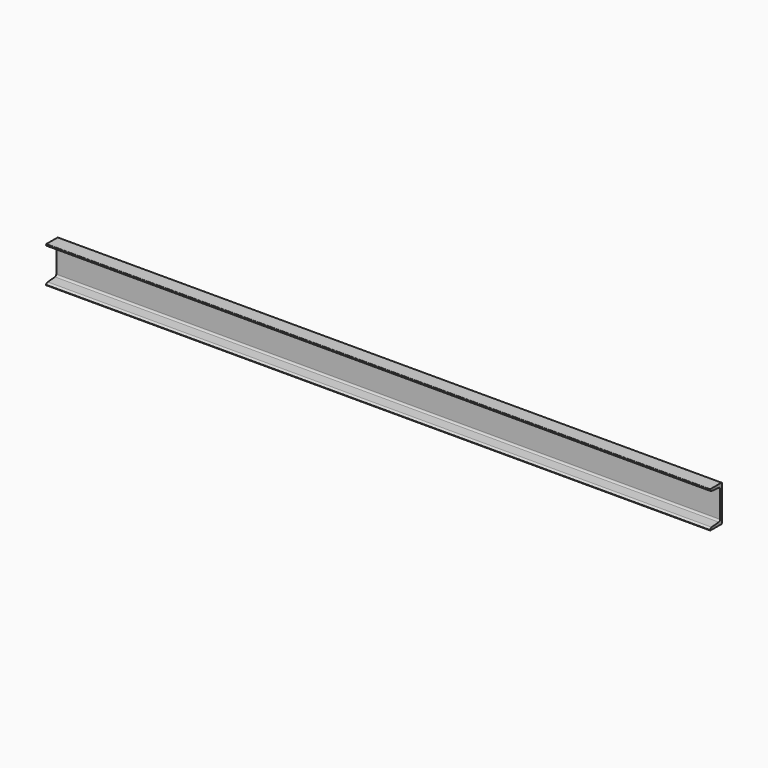
from build123d import *

# Parameters (mm, degrees)
F1_DEPTH    = 924
F2_T1_DEPTH = 1877.7738168108


# Not quite as in the source:
# - a fillet or chamfer that OpenCascade refuses, or shapes differently, is made with other operations: its cross-section is extruded or revolved along the edge and cut away or added


with BuildPart() as f1:
    # F0 (on Right) → F1 (new body, symmetric)
    with BuildSketch(Plane.YZ):
        with BuildLine():
            ThreePointArc((-20.915, -48.8), (-20.3292135624, -50.2142135624), (-18.915, -50.8))
            Line((-18.915, -50.8), (18.915, -50.8))
            ThreePointArc((18.915, -50.8), (20.3292135624, -50.2142135624), (20.915, -48.8))
            Line((20.915, -48.8), (20.915, 48.8))
            ThreePointArc((20.915, 48.8), (20.3292135624, 50.2142135624), (18.915, 50.8))
            Line((18.915, 50.8), (-18.915, 50.8))
            ThreePointArc((-18.915, 50.8), (-20.3292135624, 50.2142135624), (-20.915, 48.8))
            Line((-20.915, 48.8), (-20.915, 44.8355484375))
            Line((-20.915, 44.8355484375), (10.0807787137, 42.1237691829))
            ThreePointArc((10.0807787137, 42.1237691829), (13.3313866841, 40.5207467305), (14.645, 37.1427956924))
            Line((14.645, 37.1427956924), (14.645, -37.1427956924))
            ThreePointArc((14.645, -37.1427956924), (13.3313866841, -40.5207467305), (10.0807787137, -42.1237691829))
            Line((10.0807787137, -42.1237691829), (-20.915, -44.8355484375))
            Line((-20.915, -44.8355484375), (-20.915, -48.8))
        make_face()
    extrude(amount=F1_DEPTH, both=True)

    # F2: fillet of radius 7 on 2 edges, made by hand

    # F2_s2 → F2_t1 (cut)
    with BuildSketch(Plane.YZ.offset(-938.8869084054)):
        with BuildLine():
            ThreePointArc((-20.915, -48.8), (-18.5934823683, -45.7054865005), (-14.9828963102, -44.3165566138))
            Line((-14.9828963102, -44.3165566138), (-14.9950981142, -44.177089356))
            Line((-14.9950981142, -44.177089356), (-20.927201804, -44.6960811798))
            Line((-20.927201804, -44.6960811798), (-21.055, -44.8355484375))
            ThreePointArc((-21.055, -44.8355484375), (-21.055, -46.8177742187), (-21.0458438778, -48.75020161))
            Line((-21.0458438778, -48.75020161), (-20.915, -48.8))
        make_face()
        with BuildLine():
            ThreePointArc((-14.9828963102, 44.3165566138), (-18.5934823683, 45.7054865005), (-20.915, 48.8))
            Line((-20.915, 48.8), (-21.0458438778, 48.75020161))
            ThreePointArc((-21.0458438778, 48.75020161), (-21.055, 46.8177742187), (-21.055, 44.8355484375))
            Line((-21.055, 44.8355484375), (-20.927201804, 44.6960811798))
            Line((-20.927201804, 44.6960811798), (-14.9950981142, 44.177089356))
            Line((-14.9950981142, 44.177089356), (-14.9828963102, 44.3165566138))
        make_face()
    extrude(amount=F2_T1_DEPTH, mode=Mode.SUBTRACT)


solid = f1.part
